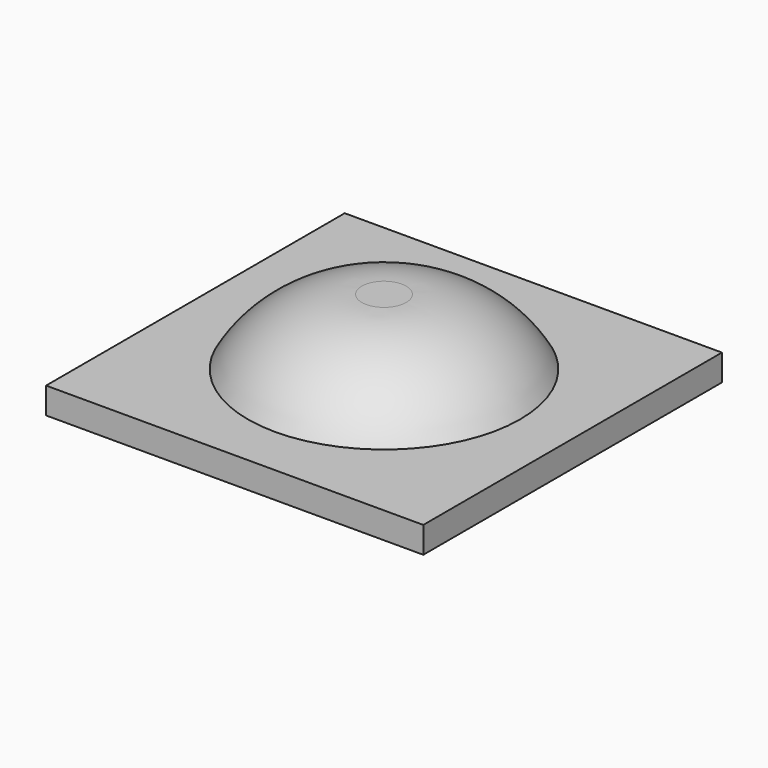
from build123d import *

# Parameters (mm, degrees)
F0_R     = 26.2781927152
F1_DEPTH = 12.7
F3_W     = 72.8053152561
F3_H     = 72.0469206572
F4_DEPTH = 5.08


# Not quite as in the source:
# - a fillet or chamfer that OpenCascade refuses, or shapes differently, is made with other operations: its cross-section is extruded or revolved along the edge and cut away or added


with BuildPart() as f1:
    # F0 (on Top) → F1 (new body)
    with BuildSketch(Plane.XY):
        Circle(F0_R)
    extrude(amount=F1_DEPTH)

    # F2: fillet of radius 25.4 on 1 edges, made by hand

    # F2_s1 → F2_t2 (revolve, cut)
    with BuildSketch(Plane.XZ):
        with BuildLine():
            ThreePointArc((26.2781927152, 0), (16.9811474591, 9.2970452561), (4.2811474591, 12.7))
            Line((4.2811474591, 12.7), (26.2781927152, 12.7))
            Line((26.2781927152, 12.7), (26.2781927152, 0))
        make_face()
    revolve(axis=Axis((0, 0, 12.7), (0, 0, 1)), mode=Mode.SUBTRACT)

    # F3 (on Top) → F4 (join)
    with BuildSketch(Plane.XY):
        Rectangle(F3_W, F3_H)
    extrude(amount=-F4_DEPTH)


solid = f1.part
